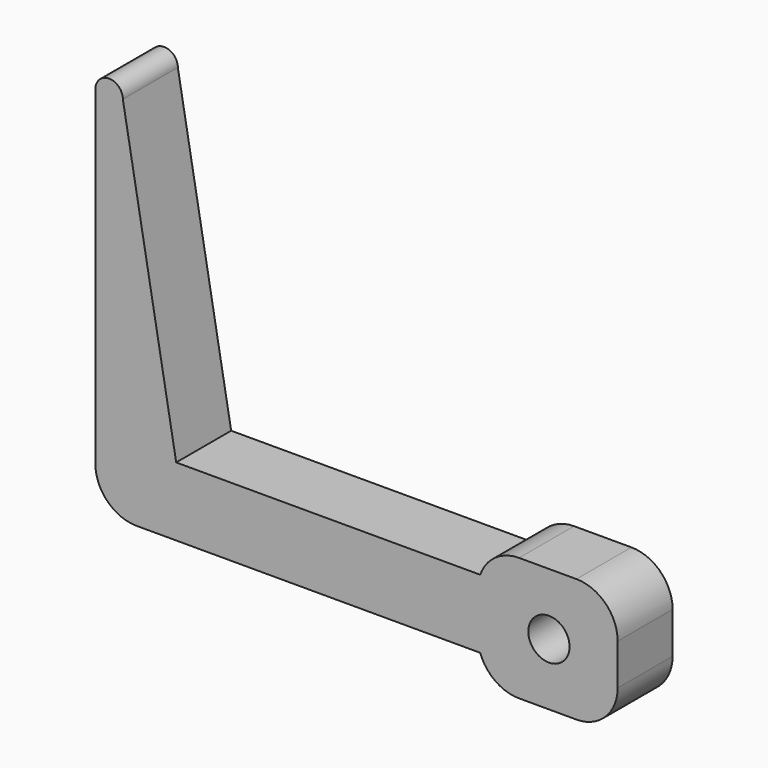
from build123d import *

# Parameters (mm, degrees)
F0_R        = 1.5
F1_DEPTH    = 5
F2_T1_DEPTH = 20
F2_T3_DEPTH = 19.1421356237


# Not quite as in the source:
# - a fillet or chamfer that OpenCascade refuses, or shapes differently, is made with other operations: its cross-section is extruded or revolved along the edge and cut away or added


with BuildPart() as f1:
    # F0 (on Front) → F1 (new body)
    with BuildSketch(Plane.XZ):
        with BuildLine():
            Line((-38, 0), (-10, 0))
            Line((-10, 0), (-10, -2))
            Line((-10, -2), (0, -2))
            Line((0, -2), (0, 0))
            Line((0, 0), (0, 5))
            Line((0, 5), (0, 7))
            Line((0, 7), (-10, 7))
            Line((-10, 7), (-10, 5))
            Line((-10, 5), (-32.1208064244, 5))
            Line((-32.1208064244, 5), (-36, 27))
            ThreePointArc((-36, 27), (-37, 28), (-38, 27))
            Line((-38, 27), (-38, 0))
        make_face()
        with Locations((-5, 2.5)):
            Circle(F0_R, mode=Mode.SUBTRACT)
    extrude(amount=F1_DEPTH)

    # F2: fillet of radius 3 on 5 edges, made by hand

    # F2_s2 → F2_t1 (cut)
    with BuildSketch(Plane.XZ.offset(-7.5)):
        with BuildLine():
            ThreePointArc((-3, 7), (-0.8786796564, 6.1213203436), (0, 4))
            Line((0, 4), (0, 7))
            Line((0, 7), (-3, 7))
        make_face()
        with BuildLine():
            ThreePointArc((0, 1), (-0.8786796564, -1.1213203436), (-3, -2))
            Line((-3, -2), (0, -2))
            Line((0, -2), (0, 1))
        make_face()
        with BuildLine():
            ThreePointArc((-35, 0), (-37.1213203436, 0.8786796564), (-38, 3))
            Line((-38, 3), (-38, 0))
            Line((-38, 0), (-35, 0))
        make_face()
    extrude(amount=F2_T1_DEPTH, mode=Mode.SUBTRACT)

    # F2_s4 → F2_t3 (cut)
    with BuildSketch(Plane.XZ.offset(-7.0710678119)):
        with BuildLine():
            ThreePointArc((-10, 5), (-8.9036236828, 6.4494897428), (-7.1715728753, 7))
            Line((-7.1715728753, 7), (-10, 7))
            Line((-10, 7), (-10, 5))
        make_face()
        with BuildLine():
            ThreePointArc((-7.1715728753, -2), (-8.9036236828, -1.4494897428), (-10, 0))
            Line((-10, 0), (-10, -2))
            Line((-10, -2), (-7.1715728753, -2))
        make_face()
    extrude(amount=F2_T3_DEPTH, mode=Mode.SUBTRACT)


solid = f1.part
